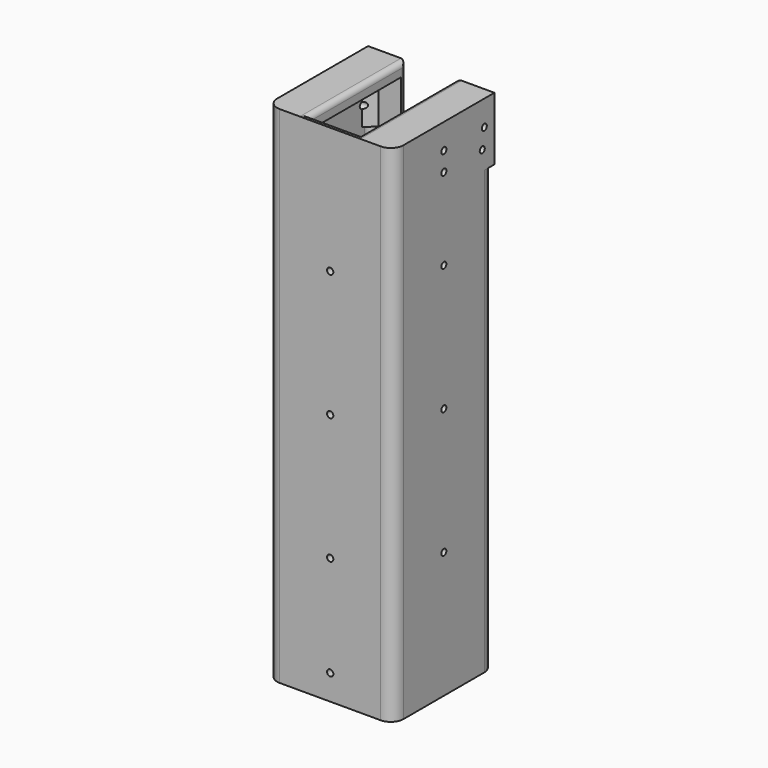
from build123d import *

# Parameters (mm, degrees)
F1_DEPTH      = 254
F1_DEPTH_BACK = 254
F4_DEPTH      = 12.7
F6_D          = 6.35
F8_D          = 6.35
F8_DEPTH      = 12.7
F8_TIP        = 1.9077324654
F10_D         = 6.35
F12_D         = 6.35
F14_DEPTH     = 25.4
F15_R         = 5.08
F17_DEPTH     = 63.5
F19_D         = 6.35
F19_DEPTH     = 12.7
F19_TIP       = 1.9077324654


# Not quite as in the source:
# - a pattern or mirror of a feature is missing from the dataset's text; its kind, count and spacing are read off the source's solid
# - a feature names something its author has since deleted; it is built from what else it names


with BuildPart() as f1:
    # F0 (on Top) → F1 (new body, two sides)
    with BuildSketch(Plane.XY) as f1_sk:
        with BuildLine():
            Line((-50.8, -63.5), (50.8, -63.5))
            ThreePointArc((50.8, -63.5), (59.7802561211, -59.7802561211), (63.5, -50.8))
            Line((63.5, -50.8), (63.5, 50.8))
            ThreePointArc((63.5, 50.8), (59.7802561211, 59.7802561211), (50.8, 63.5))
            Line((50.8, 63.5), (-50.8, 63.5))
            ThreePointArc((-50.8, 63.5), (-59.7802561211, 59.7802561211), (-63.5, 50.8))
            Line((-63.5, 50.8), (-63.5, -50.8))
            ThreePointArc((-63.5, -50.8), (-59.7802561211, -59.7802561211), (-50.8, -63.5))
        make_face()
        with BuildLine():
            ThreePointArc((50.8, 57.1499988437), (55.2901272429, 55.2901272429), (57.1499988437, 50.8))
            Line((57.1499988437, 50.8), (57.1499988437, -50.8))
            ThreePointArc((57.1499988437, -50.8), (55.2901272429, -55.2901272429), (50.8, -57.1499988437))
            Line((50.8, -57.1499988437), (-50.8, -57.1499988437))
            ThreePointArc((-50.8, -57.1499988437), (-55.2901272429, -55.2901272429), (-57.1499988437, -50.8))
            Line((-57.1499988437, -50.8), (-57.1499988437, 50.8))
            ThreePointArc((-57.1499988437, 50.8), (-55.2901272429, 55.2901272429), (-50.8, 57.1499988437))
            Line((-50.8, 57.1499988437), (50.8, 57.1499988437))
        make_face(mode=Mode.SUBTRACT)
    extrude(amount=F1_DEPTH)
    extrude(f1_sk.sketch, amount=-F1_DEPTH_BACK)

    # F3 (on face) → F4 (join)
    with BuildSketch(Plane.XY.offset(254)):
        with BuildLine():
            Line((50.8, 57.1499988437), (25.4, 57.1499988437))
            Line((25.4, 57.1499988437), (25.4, -57.1499988437))
            Line((25.4, -57.1499988437), (50.8, -57.1499988437))
            ThreePointArc((50.8, -57.1499988437), (55.2901272429, -55.2901272429), (57.1499988437, -50.8))
            Line((57.1499988437, -50.8), (57.1499988437, 50.8))
            ThreePointArc((57.1499988437, 50.8), (55.2901272429, 55.2901272429), (50.8, 57.1499988437))
        make_face()
        with BuildLine():
            Line((-25.4, -57.1499988437), (-25.4, 57.1499988437))
            Line((-25.4, 57.1499988437), (-50.8, 57.1499988437))
            ThreePointArc((-50.8, 57.1499988437), (-55.2901272429, 55.2901272429), (-57.1499988437, 50.8))
            Line((-57.1499988437, 50.8), (-57.1499988437, -50.8))
            ThreePointArc((-57.1499988437, -50.8), (-55.2901272429, -55.2901272429), (-50.8, -57.1499988437))
            Line((-50.8, -57.1499988437), (-25.4, -57.1499988437))
        make_face()
    extrude(amount=-F4_DEPTH)

    # F6 (through all)
    with Locations(Plane.YZ.offset(63.5)):
        with Locations((0, 209.55), (0, 228.6)):
            Hole(F6_D / 2)

    # F8
    with Locations(Plane.XZ.offset(63.5)):
        with Locations((0, -228.6)):
            Hole(F8_D / 2, depth=F8_DEPTH)
            with Locations((0, 0, -(F8_DEPTH + F8_TIP / 2))):  # 118° drill point
                Cone(0, F8_D / 2, F8_TIP, mode=Mode.SUBTRACT)

    # F10 (through all)
    with Locations(Plane.YZ.offset(63.5)):
        with Locations((0, 0), (0, -127), (0, 127)):
            Hole(F10_D / 2)

    # F12 (through all)
    with Locations(Plane(origin=(0, 63.5, 0), x_dir=(-1, 0, 0), z_dir=(0, 1, 0))):
        with Locations((0, 0), (0, -127), (0, 127)):
            Hole(F12_D / 2)

    # F13 (on face) → F14 (cut)
    with BuildSketch(Plane(origin=(0, 63.5, 0), x_dir=(-1, 0, 0), z_dir=(0, 1, 0))):
        with BuildLine():
            Line((25.4, 196.85), (25.4, 254))
            Line((25.4, 254), (-25.4, 254))
            Line((-25.4, 254), (-25.4, 196.85))
            ThreePointArc((-25.4, 196.85), (-23.5401280605, 192.3598719395), (-19.05, 190.5))
            Line((-19.05, 190.5), (19.05, 190.5))
            ThreePointArc((19.05, 190.5), (23.5401280605, 192.3598719395), (25.4, 196.85))
        make_face()
    extrude(amount=-F14_DEPTH, mode=Mode.SUBTRACT)

    # F15
    f15_edges = [f1.edges().sort_by_distance(p)[0] for p in [
        (25.4, 63.5, 225.425),
        (-25.4, 3.175001, 254),
        (25.4, 3.175001, 254),
        (0, -57.149999, 254),
        (-25.4, 63.5, 225.425),
        (-23.540128, 63.5, 192.359872),
        (0, 63.5, 190.5),
        (23.540128, 63.5, 192.359872),
    ]]
    fillet(f15_edges, radius=F15_R)

    # F16 (on face) → F17 (join)
    with BuildSketch(Plane.XY.offset(254)):
        with BuildLine():
            Line((-63.5, 50.8), (-63.5, 41.8197438789))
            Line((-63.5, 41.8197438789), (-41.8197438789, 63.5))
            Line((-41.8197438789, 63.5), (-50.8, 63.5))
            ThreePointArc((-50.8, 63.5), (-59.7802561211, 59.7802561211), (-63.5, 50.8))
        make_face()
        with BuildLine():
            Line((-63.5, 63.5), (-63.5, 50.8))
            ThreePointArc((-63.5, 50.8), (-59.7802561211, 59.7802561211), (-50.8, 63.5))
            Line((-50.8, 63.5), (-63.5, 63.5))
        make_face()
    f17 = extrude(amount=-F17_DEPTH)

    # F17_copies: F17 across plane
    add(f17.mirror(Plane(origin=(0, 0, 0), x_dir=(0, 0, 1), z_dir=(1, 0, 0))))

    # F19
    with Locations(Plane(origin=(-63.5, 0, 0), x_dir=(0, -1, 0), z_dir=(-1, 0, 0))):
        with Locations((-48.26, 209.7200926909), (-50.8, 228.6)):
            f19 = Hole(F19_D / 2, depth=F19_DEPTH)
            with Locations((0, 0, -(F19_DEPTH + F19_TIP / 2))):  # 118° drill point
                Cone(0, F19_D / 2, F19_TIP, mode=Mode.SUBTRACT)

    # F19_copies: F19 across plane
    add(f19.mirror(Plane(origin=(-1e-06, 0, 0), x_dir=(0, 0, 1), z_dir=(1, 0, 0))), mode=Mode.SUBTRACT)


solid = f1.part
